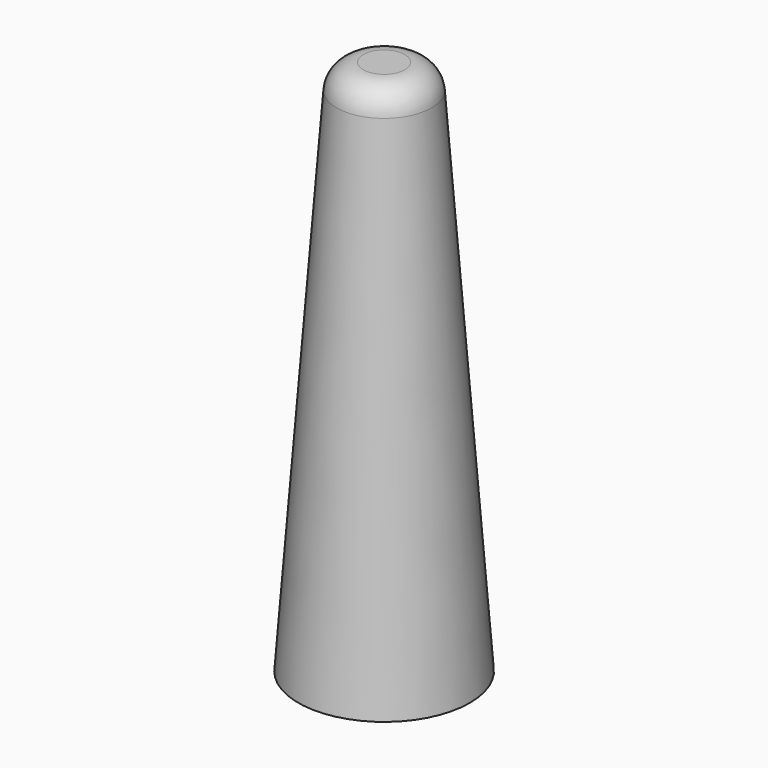
from build123d import *

# Parameters (mm, degrees)
F0_R = 3.2
F2_R = 1.7
F4_T = -1
F5_R = 1


with BuildPart() as f3:
    # F0 (on Top) → F3 section 0
    with BuildSketch(Plane.XY):
        Circle(F0_R)
    # F2 (on offset) → F3 section 1
    with BuildSketch(Plane.XY.offset(20)):
        Circle(F2_R)
    loft()

    # F4
    f4_openings = [f3.faces().sort_by_distance(p)[0] for p in [
        (0, 0, 0),
    ]]
    offset(amount=F4_T, openings=f4_openings, kind=Kind.INTERSECTION)

    # F5
    f5_edges = [f3.edges().sort_by_distance(p)[0] for p in [
        (-1.7, 0, 20),
    ]]
    fillet(f5_edges, radius=F5_R)


solid = f3.part
